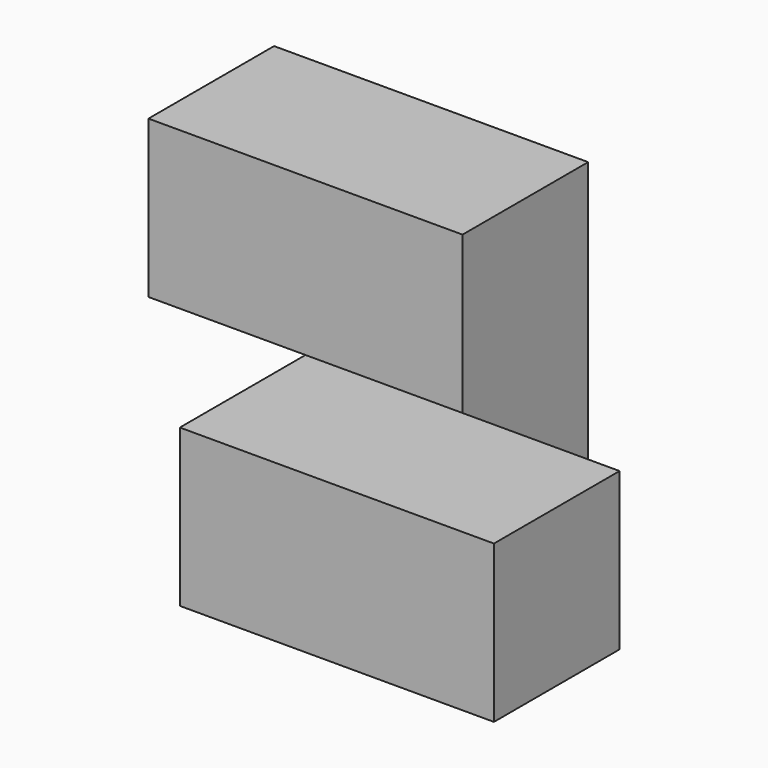
from build123d import *

# Parameters (mm, degrees)
F1_W      = 101.6
F1_H      = 101.6
F2_DEPTH  = 50.8
F3_W      = 101.6
F3_H      = 101.6
F4_DEPTH  = 101.6
F5_W      = 101.6
F5_H      = 101.6
F6_DEPTH  = 101.6
F7_W      = 101.6
F7_H      = 101.6
F8_DEPTH  = 101.6
F9_W      = 101.6
F9_H      = 101.6
F10_DEPTH = 101.6


# Not quite as in the source:
# - a variable given as a bare number and used for a length is read in inches; the dataset says mm whatever the document's units were


with BuildPart() as f2:
    # F1 (on Front) → F2 (new body, symmetric)
    with BuildSketch(Plane.XZ):
        Rectangle(F1_W, F1_H)
    extrude(amount=F2_DEPTH, both=True)

    # F3 (on face) → F4 (join)
    with BuildSketch(Plane.XZ.offset(50.8)):
        Rectangle(F3_W, F3_H)
    extrude(amount=F4_DEPTH)

    # F5 (on face) → F6 (join)
    with BuildSketch(Plane.YZ.offset(50.8)):
        with Locations((-101.6, 0)):
            Rectangle(F5_W, F5_H)
    extrude(amount=F6_DEPTH)

    # F7 (on face) → F8 (join)
    with BuildSketch(Plane.XY.offset(50.8)):
        Rectangle(F7_W, F7_H)
    extrude(amount=F8_DEPTH)

    # F9 (on face) → F10 (join)
    with BuildSketch(Plane(origin=(-50.8, 0, 0), x_dir=(0, -1, 0), z_dir=(-1, 0, 0))):
        with Locations((0, 101.6)):
            Rectangle(F9_W, F9_H)
    extrude(amount=F10_DEPTH)


solid = f2.part
